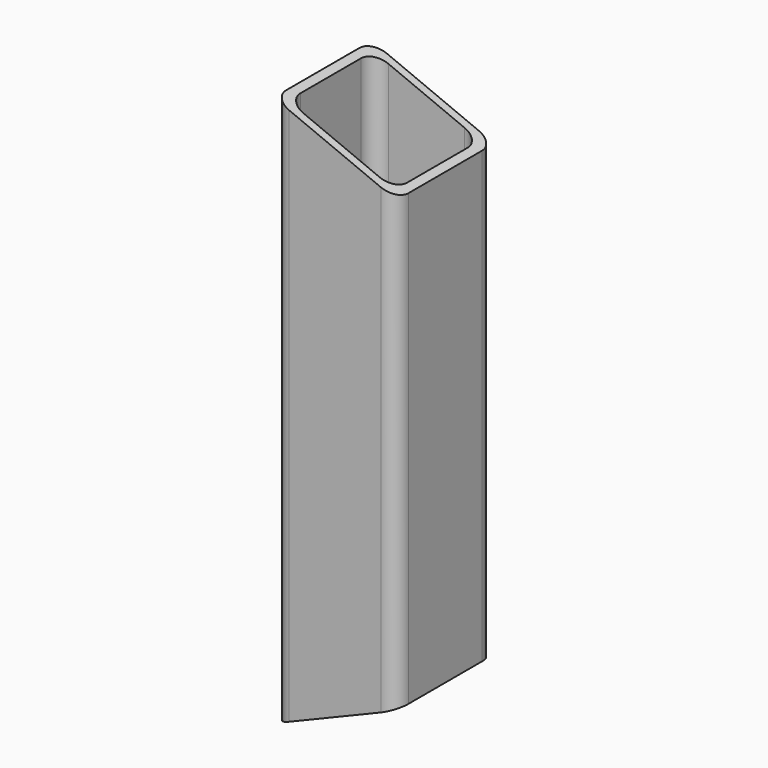
from build123d import *

# Parameters (mm, degrees)
F1_W     = 25.4
F1_H     = 25.4
F2_DEPTH = 114.3
F4_DEPTH = 25.4
F5_R     = 3.175


# Not quite as in the source:
# - a variable given as a bare number and used for a length is read in inches; the dataset says mm whatever the document's units were


with BuildPart() as f2:
    # F1 (on Top) → F2 (new body)
    with BuildSketch(Plane.XY):
        Rectangle(F1_W, F1_H)
        with BuildLine():
            ThreePointArc((-11.049, 7.874), (-10.1190640303, 10.1190640303), (-7.874, 11.049))
            Line((-7.874, 11.049), (7.874, 11.049))
            ThreePointArc((7.874, 11.049), (10.1190640303, 10.1190640303), (11.049, 7.874))
            Line((11.049, 7.874), (11.049, -7.874))
            ThreePointArc((11.049, -7.874), (10.1190640303, -10.1190640303), (7.874, -11.049))
            Line((7.874, -11.049), (-7.874, -11.049))
            ThreePointArc((-7.874, -11.049), (-10.1190640303, -10.1190640303), (-11.049, -7.874))
            Line((-11.049, -7.874), (-11.049, 7.874))
        make_face(mode=Mode.SUBTRACT)
    extrude(amount=F2_DEPTH)

    # F3 (on face) → F4 (cut)
    with BuildSketch(Plane.XZ.offset(12.7)):
        Polygon((12.7, 10.5210244843), (-12.7, 0), (12.7, 0), align=None)
        Polygon((12.7, 114.3), (-12.7, 114.3), (12.7, 103.7789755157), align=None)
    extrude(amount=-F4_DEPTH, mode=Mode.SUBTRACT)

    # F5
    f5_edges = [f2.edges().sort_by_distance(p)[0] for p in [
        (-12.7, 12.7, 57.15),
        (12.7, 12.7, 57.15),
        (-12.7, -12.7, 57.15),
        (12.7, -12.7, 57.15),
    ]]
    fillet(f5_edges, radius=F5_R)


solid = f2.part
